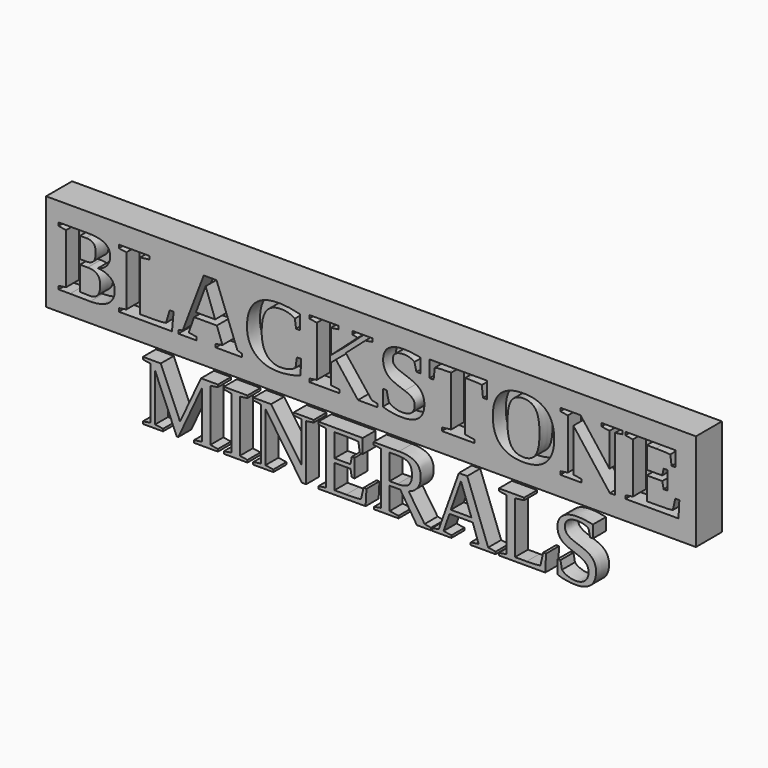
from build123d import *

# Parameters (mm, degrees)
F0_W         = 1000
F0_H         = 150
F1_DEPTH     = 50
F2_TEXT_SIZE = 138.8888888889
F3_DEPTH     = 25
F4_TEXT_SIZE = 138.8888888889
F5_DEPTH     = 25


# Not quite as in the source:
# - Text() gives the source's letters only with a copy of the font that has no kerning and outlines rounded to 1/6400 em; it was checked with that copy


with BuildPart() as f1:
    # F0 (on Front) → F1 (new body)
    with BuildSketch(Plane.XZ):
        with Locations((0, 65)):
            Rectangle(F0_W, F0_H)
    extrude(amount=-F1_DEPTH)

    # F2 (on Front) → F3 (cut)
    with BuildSketch(Plane.XZ):
        with Locations((-483.1705729167, 20)):
            Text('BLACKSTONE', F2_TEXT_SIZE, font='Tinos', font_style=FontStyle.BOLD, text_align=(TextAlign.LEFT, TextAlign.BOTTOM))
    extrude(amount=-F3_DEPTH, mode=Mode.SUBTRACT)


with BuildPart() as f5:
    # F4 (on Front) → F5 (new body)
    with BuildSketch(Plane.XZ):
        with Locations((-354.9913194444, -120)):
            Text('MINERALS', F4_TEXT_SIZE, font='Tinos', text_align=(TextAlign.LEFT, TextAlign.BOTTOM))
    extrude(amount=-F5_DEPTH)


solid = Compound([f1.part, f5.part])
